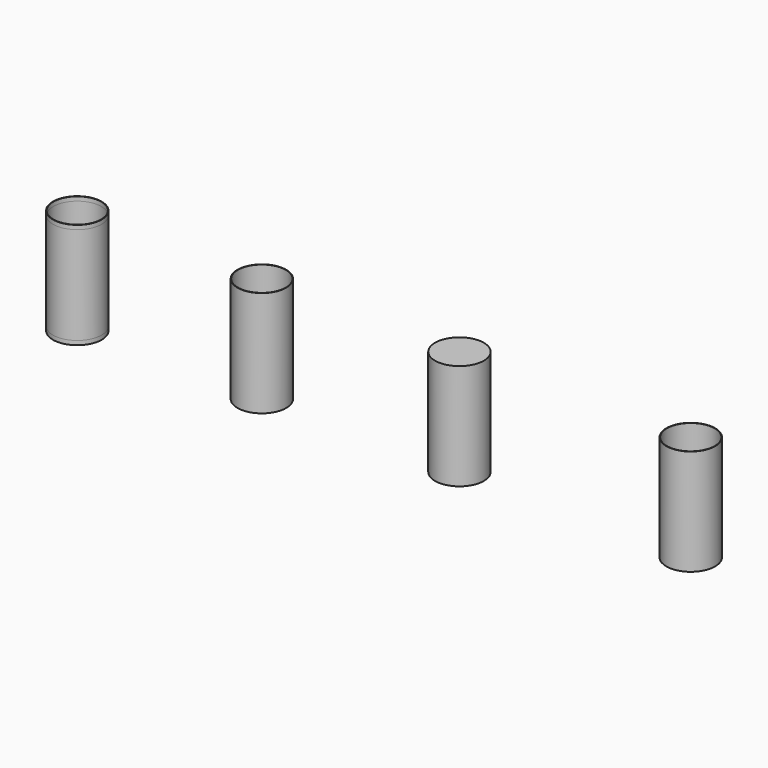
from build123d import *

# Parameters (mm, degrees)
F0_R     = 23.01875
F0_R_2   = 22.621875
F1_DEPTH = 3.9375
F2_W     = 0.396875
F2_H     = 100.0125
F5_R     = 23.01875
F5_R_2   = 22.8203125
F7_R     = 23.01875
F7_R_2   = 22.621875
F8_DEPTH = 100.0125


# Not quite as in the source:
# - a pattern or mirror of a feature is missing from the dataset's text; its kind, count and spacing are read off the source's solid


with BuildPart() as f1:
    # F0 (on Top) → F1 (new body)
    with BuildSketch(Plane.XY):
        with Locations((79.9737968977, 0)):
            Circle(F0_R)
        with Locations((79.9737968977, 0)):
            Circle(F0_R_2, mode=Mode.SUBTRACT)
    extrude(amount=F1_DEPTH)


with BuildPart() as f1_copies_1:
    # F1_copies: instance of F1
    add(f1.part.mirror(Plane.XY.offset(50.00625)))


with BuildPart() as f3:
    # F2 (on Front) → F3 (revolve)
    with BuildSketch(Plane.XZ):
        with Locations((277.110565424, 50.00625)):
            Rectangle(F2_W, F2_H)
    revolve(axis=Axis((254.290252924, 0, 67.7974149585), (0, 0, 1)))


with BuildPart() as f1_1:
    add(f1.part)

    add(f1_copies_1.part)  # F3_copies merges F1_copies_1
    # F3_copies: F3 across plane
    add(f3.part.mirror(Plane(origin=(167.132025, 0, 0), x_dir=(0, 0, -1), z_dir=(-1, 0, 0))))


with BuildPart() as f6:
    # F6: sweep along a path in F4
    with BuildLine(Plane.XZ) as f6_path:
        Line((440.9259481555, 0), (440.9259481555, 100.0125))
    # F5 (on Top) → F6 (sweep)
    with BuildSketch(Plane.XY):
        with Locations((440.9259481555, 0)):
            Circle(F5_R)
        with Locations((440.9259481555, 0)):
            Circle(F5_R_2, mode=Mode.SUBTRACT)
        with Locations((440.9259481555, 0)):
            Circle(F5_R_2)
    sweep(path=f6_path.line)


with BuildPart() as f8:
    # F7 (on Top) → F8 (new body)
    with BuildSketch(Plane.XY):
        with Locations((659.4147582325, 0)):
            Circle(F7_R)
        with Locations((659.4147582325, 0)):
            Circle(F7_R_2, mode=Mode.SUBTRACT)
    extrude(amount=F8_DEPTH)


solid = Compound([f3.part, f1_1.part, f6.part, f8.part])
